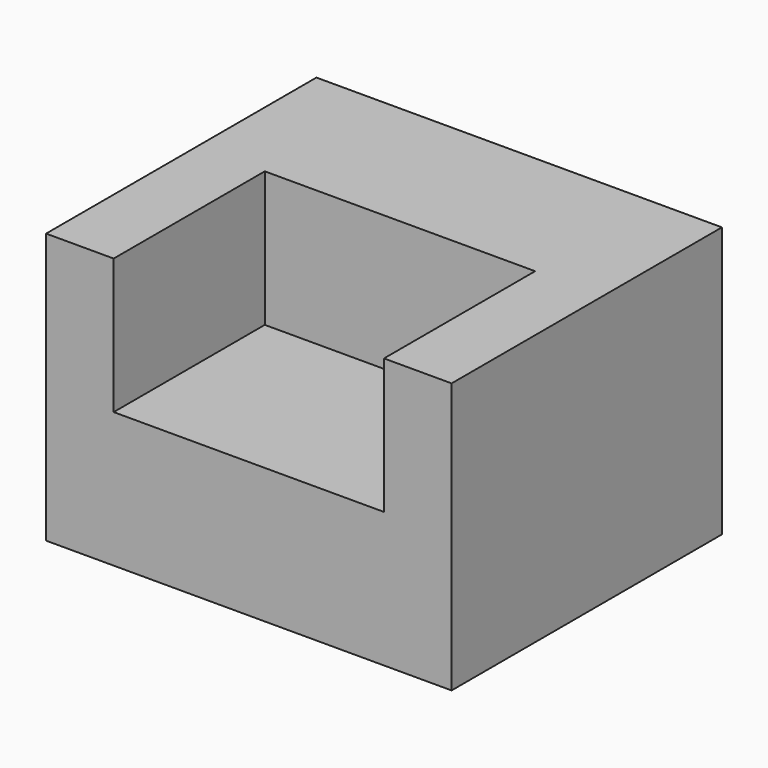
from build123d import *

# Parameters (mm, degrees)
F1_DEPTH = 127
F2_W     = 101.6
F2_H     = 56.0078546405
F3_DEPTH = 50.8


with BuildPart() as f1:
    # F0 (on Front) → F1 (new body)
    with BuildSketch(Plane.XZ):
        Polygon((-104.5768260956, 64.1456519425), (-104.5768260956, -37.4543480575), (47.8231739044, -37.4543480575), (47.8231739044, 64.1456519425), (22.4231739044, 64.1456519425), (22.4231739044, 13.3456519425), (-79.1768260956, 13.3456519425), (-79.1768260956, 64.1456519425), align=None)
    extrude(amount=F1_DEPTH)

    # F2 (on face) → F3 (join)
    with BuildSketch(Plane.XY.offset(13.3456519425)):
        with Locations((-28.3768260956, -28.0039273202)):
            Rectangle(F2_W, F2_H)
    extrude(amount=F3_DEPTH)


solid = f1.part
